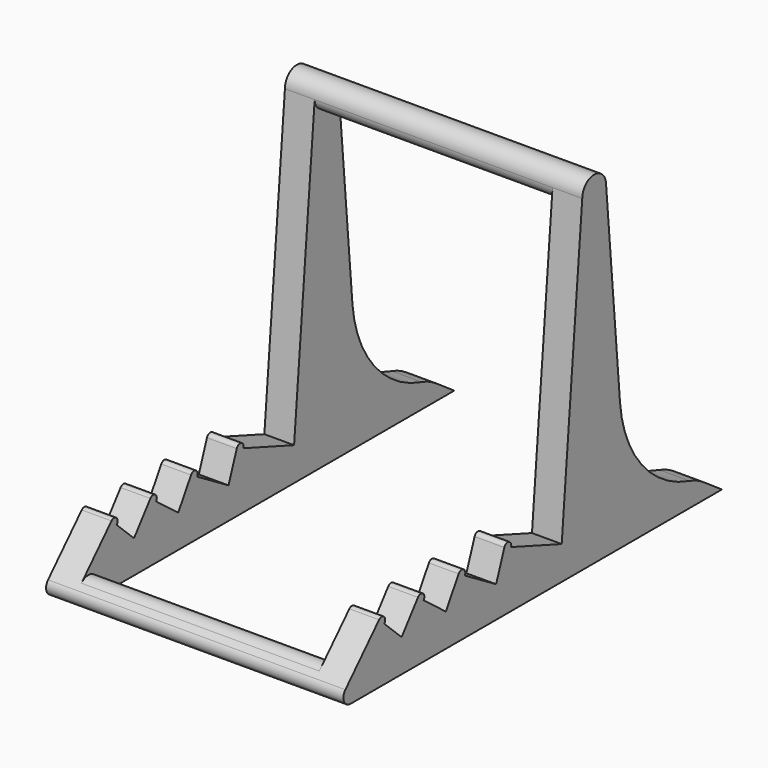
from build123d import *

# Parameters (mm, degrees)
F1_DEPTH      = 25
F1_DEPTH_BACK = 25
F2_W          = 40
F2_H          = 55.1616017345
F3_DEPTH      = 55
F3_DEPTH_BACK = 25
F4_T1_DEPTH   = 40
F5_R          = 1.5
F6_T1_DEPTH   = 5
F6_T3_DEPTH   = 5
F6_T8_DEPTH   = 86.3985693966
F6_T13_DEPTH  = 86.3985693966
F7_T1_DEPTH   = 14.1895410393
F7_T3_DEPTH   = 14.1895410393


# Not quite as in the source:
# - a fillet or chamfer that OpenCascade refuses, or shapes differently, is made with other operations: its cross-section is extruded or revolved along the edge and cut away or added
# - two fillets or chamfers of one size are made in one step


with BuildPart() as f1:
    # F0 (on Right) → F1 (new body, two sides)
    with BuildSketch(Plane.YZ) as f1_sk:
        with BuildLine():
            Line((44.6048974991, -1.3002553023), (30, 0.3549050016))
            Line((30, 0.3549050016), (25.6348953616, 50.2482793254))
            ThreePointArc((25.6348953616, 50.2482793254), (23.0201813599, 52.5273015786), (20.6445933332, 50))
            Line((20.6445933332, 50), (16.7076034746, 5))
            Line((16.7076034746, 5), (16.3236464507, 0.6113511347))
            Line((16.3236464507, 0.6113511347), (5.6754717224, 4.486969785))
            Line((5.6754717224, 4.486969785), (4.2659327913, 5))
            Line((4.2659327913, 5), (2.5413501994, 0.2617482709))
            Line((2.5413501994, 0.2617482709), (-4.0507753245, 4.2268482272))
            Line((-4.0507753245, 4.2268482272), (-5.3361687803, 5))
            Line((-5.3361687803, 5), (-8.0358432445, 0.5116912215))
            Line((-8.0358432445, 0.5116912215), (-12.6950911154, 4.0868578565))
            Line((-12.6950911154, 4.0868578565), (-13.8851211258, 5))
            Line((-13.8851211258, 5), (-17.329121582, 0.5116912215))
            Line((-17.329121582, 0.5116912215), (-20.9707506124, 3.9674681365))
            Line((-20.9707506124, 3.9674681365), (-22.0588121689, 5))
            Line((-22.0588121689, 5), (-31.5484578361, -5))
            Line((-31.5484578361, -5), (50, -5))
            Line((50, -5), (44.6048974991, -1.3002553023))
        make_face()
        with BuildLine():
            ThreePointArc((-20.9707506124, 3.9674681365), (-20.9985154589, 5.0277648465), (-22.0588121689, 5))
            Line((-22.0588121689, 5), (-20.9707506124, 3.9674681365))
        make_face()
        with BuildLine():
            Line((4.2659327913, 5), (5.6754717224, 4.486969785))
            ThreePointArc((5.6754717224, 4.486969785), (5.2272173643, 5.4482543581), (4.2659327913, 5))
        make_face()
        with BuildLine():
            ThreePointArc((-12.6950911154, 4.0868578565), (-12.8335350488, 5.1384439335), (-13.8851211258, 5))
            Line((-13.8851211258, 5), (-12.6950911154, 4.0868578565))
        make_face()
        with BuildLine():
            Line((-5.3361687803, 5), (-4.0507753245, 4.2268482272))
            ThreePointArc((-4.0507753245, 4.2268482272), (-4.306896166, 5.2561208415), (-5.3361687803, 5))
        make_face()
    extrude(amount=F1_DEPTH)
    extrude(f1_sk.sketch, amount=-F1_DEPTH_BACK)

    # F2 (on face) → F3 (cut, two sides)
    with BuildSketch(Plane(origin=(0, 29.8029305986, 2.6074185672), x_dir=(-1, 0, 0), z_dir=(0, 0.9961946981, 0.0871557427))) as f3_sk:
        with Locations((0, 18.2420402394)):
            Rectangle(F2_W, F2_H)
    extrude(amount=-F3_DEPTH, mode=Mode.SUBTRACT)
    extrude(f3_sk.sketch, amount=F3_DEPTH_BACK, mode=Mode.SUBTRACT)

    # F4: fillet of radius 2 on 2 edges, made by hand

    # F4_s2 → F4_t1 (cut)
    with BuildSketch(Plane.YZ.offset(-20)):
        with BuildLine():
            ThreePointArc((-24.9292183204, -2.8554851584), (-26.262226426, -1.1416186031), (-28.3723564586, -1.6530874925))
            Line((-28.3723564586, -1.6530874925), (-25.3161754694, 1.5674552932))
            Line((-25.3161754694, 1.5674552932), (-24.9292183204, -2.8554851584))
        make_face()
        with BuildLine():
            ThreePointArc((22.8188603154, 47.9942685076), (21.2884574912, 48.5166183529), (20.6445933332, 50))
            Line((20.6445933332, 50), (20.4509902577, 47.7871067209))
            Line((20.4509902577, 47.7871067209), (22.8188603154, 47.9942685076))
        make_face()
    extrude(amount=F4_T1_DEPTH, mode=Mode.SUBTRACT)

    # F5
    f5_edges = [f1.edges().sort_by_distance(p)[0] for p in [
        (0, -31.548458, -5),
        (0, -24.741598, -5),
    ]]
    fillet(f5_edges, radius=F5_R)

    # F6: fillet of radius 20 on 2 edges, made by hand

    # F6_s2 → F6_t1 (join)
    with BuildSketch(Plane.YZ.offset(20)):
        with BuildLine():
            ThreePointArc((44.6048974991, -1.3002553023), (33.6135378425, 4.9649921105), (28.5811294451, 16.5726696546))
            Line((28.5811294451, 16.5726696546), (30, 0.3549050016))
            Line((30, 0.3549050016), (44.6048974991, -1.3002553023))
        make_face()
    extrude(amount=F6_T1_DEPTH)

    # F6_s4 → F6_t3 (join)
    with BuildSketch(Plane.YZ.offset(-25)):
        with BuildLine():
            ThreePointArc((28.5811294451, 16.5726696546), (33.6135378425, 4.9649921105), (44.6048974991, -1.3002553023))
            Line((44.6048974991, -1.3002553023), (30, 0.3549050016))
            Line((30, 0.3549050016), (28.5811294451, 16.5726696546))
        make_face()
    extrude(amount=F6_T3_DEPTH)


with BuildPart() as f6_tool6:
    # F6_s7 → F6_t8 (new body)
    with BuildSketch(Plane.YZ.offset(-20.6992846983)):
        with BuildLine():
            ThreePointArc((44.6048974991, -1.3002553023), (33.6135378425, 4.9649921105), (28.5811294451, 16.5726696546))
            Line((28.5811294451, 16.5726696546), (30, 0.3549050016))
            Line((30, 0.3549050016), (44.6048974991, -1.3002553023))
        make_face()
    extrude(amount=F6_T8_DEPTH)

    split(bisect_by=Plane.YZ.offset(-20), keep=Keep.BOTTOM)


with BuildPart() as f1_1:
    add(f1.part)

    # F6_t5: union F6_tool6
    add(f6_tool6.part)


with BuildPart() as f6_tool11:
    # F6_s12 → F6_t13 (new body)
    with BuildSketch(Plane.YZ.offset(-65.6992846983)):
        with BuildLine():
            ThreePointArc((28.5811294451, 16.5726696546), (33.6135378425, 4.9649921105), (44.6048974991, -1.3002553023))
            Line((44.6048974991, -1.3002553023), (30, 0.3549050016))
            Line((30, 0.3549050016), (28.5811294451, 16.5726696546))
        make_face()
    extrude(amount=F6_T13_DEPTH)

    split(bisect_by=Plane.YZ.offset(20), keep=Keep.TOP)


with BuildPart() as f1_2:
    add(f1_1.part)

    # F6_t10: union F6_tool11
    add(f6_tool11.part)

    # F7: fillet of radius 10 on 4 edges, made by hand

    # F7_s2 → F7_t1 (cut)
    with BuildSketch(Plane.YZ.offset(-29.5947705196)):
        with BuildLine():
            ThreePointArc((46.1206412105, -2.339691487), (44.6901693803, -1.5232068735), (43.1450758344, -0.9526083144))
            ThreePointArc((43.1450758344, -0.9526083144), (43.871724925, -1.1401283494), (44.6048974991, -1.3002553023))
            Line((44.6048974991, -1.3002553023), (46.1206412105, -2.339691487))
        make_face()
    extrude(amount=F7_T1_DEPTH, mode=Mode.SUBTRACT)

    # F7_s4 → F7_t3 (cut)
    with BuildSketch(Plane.YZ.offset(15.4052294804)):
        with BuildLine():
            ThreePointArc((43.1450758344, -0.9526083144), (44.6901693803, -1.5232068735), (46.1206412105, -2.339691487))
            Line((46.1206412105, -2.339691487), (44.6048974991, -1.3002553023))
            ThreePointArc((44.6048974991, -1.3002553023), (43.871724925, -1.1401283494), (43.1450758344, -0.9526083144))
        make_face()
    extrude(amount=F7_T3_DEPTH, mode=Mode.SUBTRACT)


solid = f1_2.part
